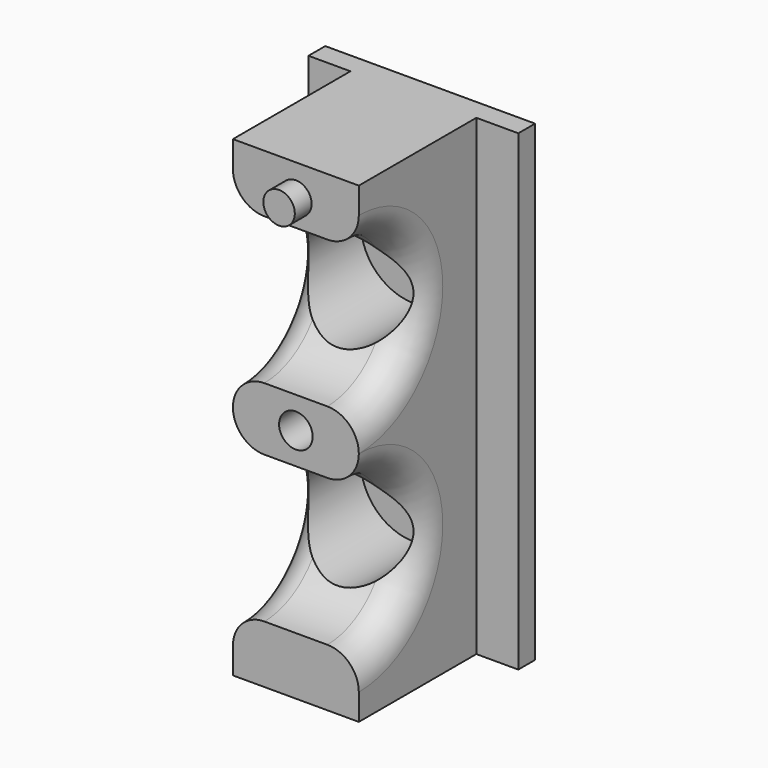
from build123d import *

# Parameters (mm, degrees)
F1_W            = 12
F1_H            = 45
F2_DEPTH        = 30
F3_R            = 7
F4_DEPTH        = 12.001
F5_W            = 20
F5_H            = 45
F6_DEPTH        = 2
F7_R            = 2.99999
F9_D            = 3.2
F11_SIZE        = 1
F13_D           = 5.1
F13_CBORE_D     = 10
F13_CBORE_DEPTH = 14
F15_DEPTH       = 5
F16_W           = 41.8421067297
F16_H           = 67.5000026822
F17_DEPTH       = 25
F18_R           = 1.5
F19_DEPTH       = 2


# Not quite as in the source:
# - a fillet or chamfer is up to 0.001 mm smaller than in the source, because OpenCascade refuses the exact size


with BuildPart() as f2:
    # F1 (on Front) → F2 (new body)
    with BuildSketch(Plane.XZ):
        Rectangle(F1_W, F1_H)
    extrude(amount=F2_DEPTH)

    # F3 (on face) → F4 (cut, through all)
    with BuildSketch(Plane.YZ.offset(6)):
        with Locations((-16, 10)):
            Circle(F3_R)
        with Locations((-16, -10)):
            Circle(F3_R)
    extrude(amount=-F4_DEPTH, mode=Mode.SUBTRACT)

    # F5 (on Front) → F6 (join)
    with BuildSketch(Plane.XZ):
        Rectangle(F5_W, F5_H)
    extrude(amount=F6_DEPTH)

    # F7 (radius 3 in the source; OpenCascade refuses exactly that, so slightly less here)
    f7_edges = [f2.edges().sort_by_distance(p)[0] for p in [
        (-6, -23, 10),
        (-6, -23, -10),
        (6, -23, 10),
        (6, -23, -10),
    ]]
    fillet(f7_edges, radius=F7_R)

    # F9 (through all)
    with Locations(Plane(origin=(0, 0, 0), x_dir=(-1, 0, 0), z_dir=(0, 1, 0))):
        with Locations((0, 10), (0, -10), (0, 0)):
            Hole(F9_D / 2)

    # F11
    f11_edges = [f2.edges().sort_by_distance(p)[0] for p in [
        (0, -30, -22.5),
        (0, -30, 22.5),
    ]]
    chamfer(f11_edges, length=F11_SIZE)

    # F13 (through all)
    with Locations(Plane.XZ.offset(16)):
        with Locations((0, -10), (0, 10)):
            CounterBoreHole(F13_D / 2, F13_CBORE_D / 2, F13_CBORE_DEPTH)

    # F14 (on face) → F15 (cut)
    with BuildSketch(Plane(origin=(0, 0, 0), x_dir=(-1, 0, 0), z_dir=(0, 1, 0))):
        Polygon((2.3094010768, -4), (4.6188021535, 0), (2.3094010768, 4), (-2.3094010768, 4), (-4.6188021535, 0), (-2.3094010768, -4), align=None)
    extrude(amount=-F15_DEPTH, mode=Mode.SUBTRACT)

    # F16 (on offset) → F17 (cut)
    with BuildSketch(Plane.XZ.offset(16)):
        with Locations((-0.493420288, -0.09868294)):
            Rectangle(F16_W, F16_H)
    extrude(amount=F17_DEPTH, mode=Mode.SUBTRACT)

    # F18 (on face) → F19 (join)
    with BuildSketch(Plane.XZ.offset(16)):
        with Locations((0, 19.5)):
            Circle(F18_R)
    extrude(amount=F19_DEPTH)


solid = f2.part
